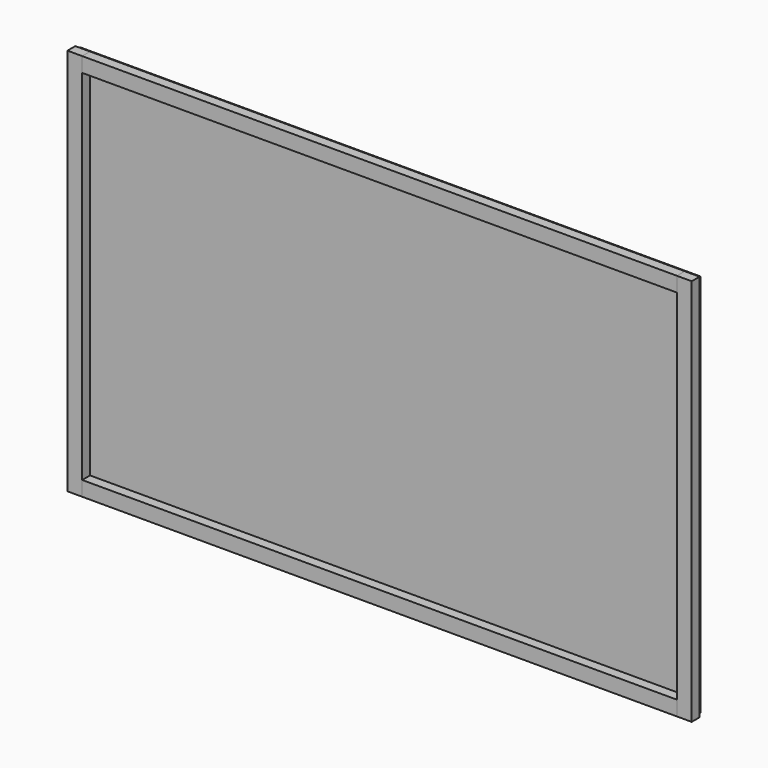
from build123d import *

# Parameters (mm, degrees)
F2_W     = 1600.2
F2_H     = 990.6
F3_DEPTH = 9.525
F5_DEPTH = 25.4
F4_W     = 1534
F4_H     = 33.1
F4_H_2   = 5
F6_DEPTH = 25.4
F7_DEPTH = 25.4
F8_DEPTH = 25.4


# Not quite as in the source:
# - a length typed as a fraction of an inch, garbled in the dataset ("3 / 203.2 mm" for 3/8 in), is restored


with BuildPart() as f3:
    # F2 (on Front) → F3 (new body)
    with BuildSketch(Plane.XZ):
        with Locations((800.1, 495.3)):
            Rectangle(F2_W, F2_H)
    extrude(amount=F3_DEPTH)


with BuildPart() as f5:
    # F4 (on face) → F5 (new body)
    with BuildSketch(Plane.XZ.offset(9.525)):
        Polygon((33.1, 957.5), (33.1, 990.6), (0, 990.6), (0, 0), (33.1, 0), (33.1, 33.1), align=None)
        Polygon((33.1, 995.6), (-5, 995.6), (-5, -5), (33.1, -5), (33.1, 0), (0, 0), (0, 990.6), (33.1, 990.6), align=None)
    extrude(amount=F5_DEPTH)


with BuildPart() as f6:
    # F4 (on face) → F6 (new body)
    with BuildSketch(Plane.XZ.offset(9.525)):
        with Locations((800.1, 974.05)):
            Rectangle(F4_W, F4_H)
        with Locations((800.1, 993.1)):
            Rectangle(F4_W, F4_H_2)
    extrude(amount=F6_DEPTH)


with BuildPart() as f7:
    # F4 (on face) → F7 (new body)
    with BuildSketch(Plane.XZ.offset(9.525)):
        Polygon((1600.2, 990.6), (1567.1, 990.6), (1567.1, 957.5), (1567.1, 33.1), (1567.1, 0), (1600.2, 0), align=None)
        Polygon((1605.2, 995.6), (1567.1, 995.6), (1567.1, 990.6), (1600.2, 990.6), (1600.2, 0), (1567.1, 0), (1567.1, -5), (1605.2, -5), align=None)
    extrude(amount=F7_DEPTH)


with BuildPart() as f8:
    # F4 (on face) → F8 (new body)
    with BuildSketch(Plane.XZ.offset(9.525)):
        with Locations((800.1, 16.55)):
            Rectangle(F4_W, F4_H)
        with Locations((800.1, -2.5)):
            Rectangle(F4_W, F4_H_2)
    extrude(amount=F8_DEPTH)


solid = Compound([f3.part, f5.part, f6.part, f7.part, f8.part])
